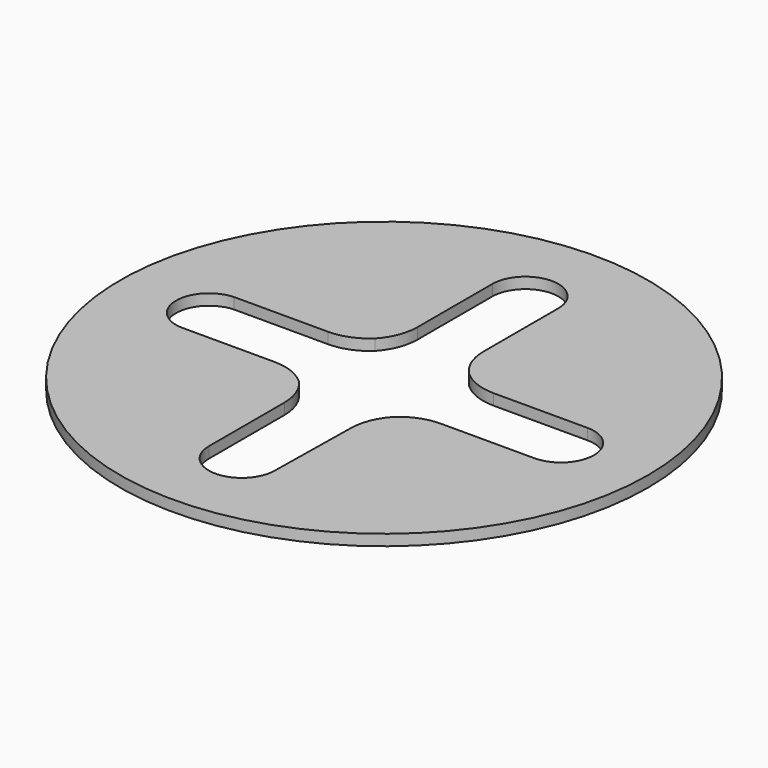
from build123d import *

# Parameters (mm, degrees)
F0_R         = 38.1
F1_DEPTH     = 1.5875
F2_T1_DEPTH  = 19.6594045054
F2_T3_DEPTH  = 19.7689044348
F2_T5_DEPTH  = 19.8002867112
F2_T7_DEPTH  = 19.8028708993
F2_T9_DEPTH  = 19.7937834769
F2_T11_DEPTH = 19.3627357335
F2_T13_DEPTH = 19.2813787557
F2_T15_DEPTH = 19.9326468644


# Not quite as in the source:
# - a fillet or chamfer that OpenCascade refuses, or shapes differently, is made with other operations: its cross-section is extruded or revolved along the edge and cut away or added


with BuildPart() as f1:
    # F0 (on Top) → F1 (new body)
    with BuildSketch(Plane.XY):
        Circle(F0_R)
        with BuildLine():
            ThreePointArc((25.5212023113, 4.7665246553), (30.2837023113, 0.0040246553), (25.5212023113, -4.7584753447))
            Line((25.5212023113, -4.7584753447), (8.3700942824, -4.7584753447))
            ThreePointArc((8.3700942824, -4.7584753447), (6.8307613912, -6.7854450641), (4.8140826203, -8.3382356902))
            Line((4.8140826203, -8.3382356902), (4.5445678914, -25.4872259938))
            ThreePointArc((4.5445678914, -25.4872259938), (-0.2648058004, -30.1554173191), (-4.9795027497, -25.3916248979))
            Line((-4.9795027497, -25.3916248979), (-4.9795027497, -8.2405168689))
            ThreePointArc((-4.9795027497, -8.2405168689), (-6.9221674375, -6.692171835), (-8.4040103572, -4.6983162748))
            Line((-8.4040103572, -4.6983162748), (-25.5551183861, -4.6983162748))
            ThreePointArc((-25.5551183861, -4.6983162748), (-30.0672979191, 0.0912532901), (-25.4878952685, 4.8165905393))
            Line((-25.4878952685, 4.8165905393), (-8.3367872396, 4.8165905393))
            ThreePointArc((-8.3367872396, 4.8165905393), (-6.7888119889, 6.8274151536), (-4.7692424862, 8.3639638934))
            Line((-4.7692424862, 8.3639638934), (-4.7692424862, 25.5150719223))
            ThreePointArc((-4.7692424862, 25.5150719223), (-0.0106390137, 30.260270074), (4.7556603142, 25.5228020557))
            Line((4.7556603142, 25.5228020557), (4.7556603142, 8.3716940268))
            ThreePointArc((4.7556603142, 8.3716940268), (6.8069974407, 6.8092842314), (8.3700961728, 4.7584720195))
            Line((8.3700961728, 4.7584720195), (25.5212023113, 4.7665246553))
        make_face(mode=Mode.SUBTRACT)
    extrude(amount=F1_DEPTH)

    # F2: fillet of radius 7.62 on 8 edges, made by hand

    # F2_s2 → F2_t1 (cut)
    with BuildSketch(Plane.XY.offset(-9.0359522527)):
        with BuildLine():
            ThreePointArc((-11.9511681406, 4.8165905393), (-9.1053172731, 5.3679603439), (-6.6713079375, 6.9422774581))
            ThreePointArc((-6.6713079375, 6.9422774581), (-7.5789423028, 5.9381141343), (-8.3367872396, 4.8165905393))
            Line((-8.3367872396, 4.8165905393), (-11.9511681406, 4.8165905393))
        make_face()
    extrude(amount=F2_T1_DEPTH, mode=Mode.SUBTRACT)

    # F2_s4 → F2_t3 (cut)
    with BuildSketch(Plane.XY.offset(-9.0907022174)):
        with BuildLine():
            ThreePointArc((-6.9158471176, 6.6987031989), (-5.3262518764, 9.1404259669), (-4.7692424862, 12.0002447803))
            Line((-4.7692424862, 12.0002447803), (-4.7692424862, 8.3639638934))
            ThreePointArc((-4.7692424862, 8.3639638934), (-5.9015763197, 7.607428136), (-6.9158471176, 6.6987031989))
        make_face()
    extrude(amount=F2_T3_DEPTH, mode=Mode.SUBTRACT)

    # F2_s6 → F2_t5 (cut)
    with BuildSketch(Plane.XY.offset(-9.1063933556)):
        with BuildLine():
            ThreePointArc((4.7556603142, 12.014251369), (5.3142882964, 9.1504383117), (6.9082653607, 6.7065218711))
            ThreePointArc((6.9082653607, 6.7065218711), (5.8910941356, 7.615548292), (4.7556603142, 8.3716940268))
            Line((4.7556603142, 8.3716940268), (4.7556603142, 12.014251369))
        make_face()
    extrude(amount=F2_T5_DEPTH, mode=Mode.SUBTRACT)

    # F2_s8 → F2_t7 (cut)
    with BuildSketch(Plane.XY.offset(-9.1076854497)):
        with BuildLine():
            ThreePointArc((6.703921101, 6.9107892294), (9.1487661341, 5.3175989867), (12.0131699511, 4.7601824833))
            Line((12.0131699511, 4.7601824833), (8.3700961728, 4.7584720195))
            ThreePointArc((8.3700961728, 4.7584720195), (7.6134497132, 5.893806017), (6.703921101, 6.9107892294))
        make_face()
    extrude(amount=F2_T7_DEPTH, mode=Mode.SUBTRACT)

    # F2_s10 → F2_t9 (cut)
    with BuildSketch(Plane.XY.offset(-9.1031417385)):
        with BuildLine():
            ThreePointArc((12.0113509777, -4.7584753447), (9.1483653066, -5.3167678283), (6.7049028325, -6.9098367498))
            ThreePointArc((6.7049028325, -6.9098367498), (7.6138671828, -5.8932667023), (8.3700942824, -4.7584753447))
            Line((8.3700942824, -4.7584753447), (12.0113509777, -4.7584753447))
        make_face()
    extrude(amount=F2_T9_DEPTH, mode=Mode.SUBTRACT)

    # F2_s12 → F2_t11 (cut)
    with BuildSketch(Plane.XY.offset(-8.8876178667)):
        with BuildLine():
            ThreePointArc((6.90916797, -6.7055919846), (5.3384286521, -9.0938512154), (4.7582181499, -11.8928438791))
            Line((4.7582181499, -11.8928438791), (4.8140826203, -8.3382356902))
            ThreePointArc((4.8140826203, -8.3382356902), (5.9181950346, -7.5945067933), (6.90916797, -6.7055919846))
        make_face()
    extrude(amount=F2_T11_DEPTH, mode=Mode.SUBTRACT)

    # F2_s14 → F2_t13 (cut)
    with BuildSketch(Plane.XY.offset(-8.8469393778)):
        with BuildLine():
            ThreePointArc((-4.9795027497, -11.7792926201), (-5.5115025024, -8.9820345887), (-7.0332173151, -6.5753646363))
            ThreePointArc((-7.0332173151, -6.5753646363), (-6.06378956, -7.478771428), (-4.9795027497, -8.2405168689))
            Line((-4.9795027497, -8.2405168689), (-4.9795027497, -11.7792926201))
        make_face()
    extrude(amount=F2_T13_DEPTH, mode=Mode.SUBTRACT)

    # F2_s16 → F2_t15 (cut)
    with BuildSketch(Plane.XY.offset(-9.1725734322)):
        with BuildLine():
            ThreePointArc((-6.7393383503, -6.8762551219), (-9.1924239959, -5.2637820597), (-12.0730397301, -4.6983162748))
            Line((-12.0730397301, -4.6983162748), (-8.4040103572, -4.6983162748))
            ThreePointArc((-8.4040103572, -4.6983162748), (-7.6495821405, -5.8468332435), (-6.7393383503, -6.8762551219))
        make_face()
    extrude(amount=F2_T15_DEPTH, mode=Mode.SUBTRACT)


solid = f1.part
